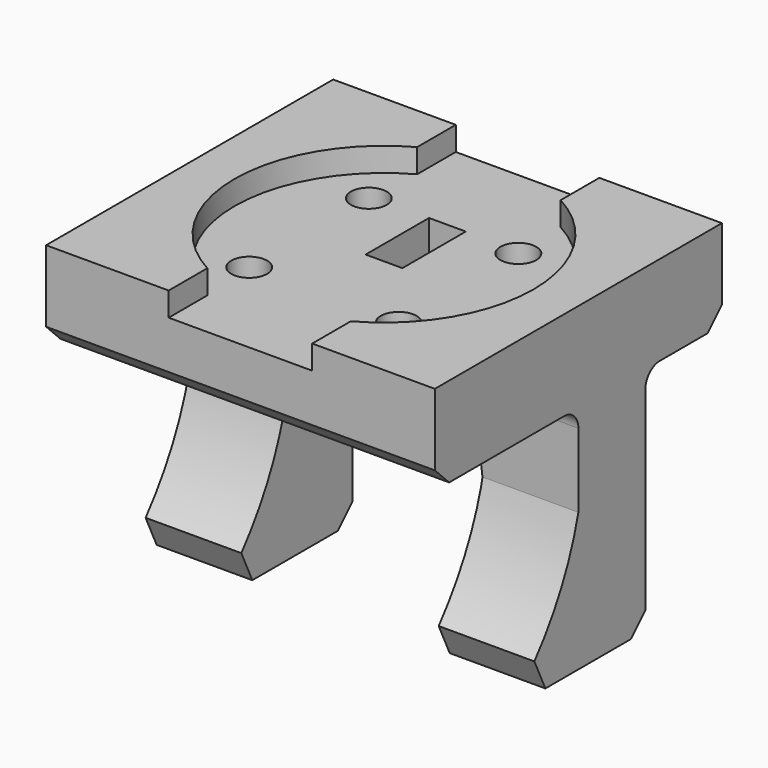
from build123d import *

# Parameters (mm, degrees)
F0_W          = 65
F0_H          = 60
F0_W_2        = 6.15
F0_H_2        = 13.25
F1_DEPTH      = 15
F3_DEPTH      = 14
F5_DEPTH      = 4
F6_R          = 3
F7_DEPTH      = 8
F9_DEPTH      = 90
F10_T4_DEPTH  = 29.425
F10_S5_R      = 16.5
F10_T6_DEPTH  = 16
F10_T10_DEPTH = 44.425
F10_S11_R     = 16.5
F10_T12_DEPTH = 24
F10_T17_DEPTH = 44.425
F10_S18_R     = 16.5
F10_T19_DEPTH = 24
F10_T24_DEPTH = 29.425
F10_S25_R     = 16.5
F10_T26_DEPTH = 16
F10_T30_DEPTH = 44.425
F10_S31_R     = 16.5
F10_T32_DEPTH = 24
F10_T37_DEPTH = 29.425
F10_S38_R     = 16.5
F10_T39_DEPTH = 16
F10_T43_DEPTH = 29.425
F10_S44_R     = 16.5
F10_T45_DEPTH = 16
F10_T49_DEPTH = 44.425
F10_S50_R     = 16.5
F10_T51_DEPTH = 24
F11_T1_DEPTH  = 80.4300979278
F11_T3_DEPTH  = 51.7830754439
F11_T5_DEPTH  = 51.7830754439
F11_T7_DEPTH  = 31.4300979278
F11_T9_DEPTH  = 31.4300979278


# Not quite as in the source:
# - a fillet or chamfer that OpenCascade refuses, or shapes differently, is made with other operations: its cross-section is extruded or revolved along the edge and cut away or added


with BuildPart() as f1:
    # F0 (on Top) → F1 (new body)
    with BuildSketch(Plane.XY):
        Rectangle(F0_W, F0_H)
        with Locations((0, 6.625)):
            Rectangle(F0_W_2, F0_H_2, mode=Mode.SUBTRACT)
    extrude(amount=F1_DEPTH)

    # F2 (on Front) → F3 (join, symmetric)
    with BuildSketch(Plane.XZ):
        with BuildLine():
            Line((-3.075, 0), (-32.5, 0))
            Line((-32.5, 0), (-32.5, -38.5))
            Line((-32.5, -38.5), (-16.5, -38.5))
            Line((-16.5, -38.5), (-16.5, -16.5))
            ThreePointArc((-16.5, -16.5), (-12.7080191218, -5.9759204678), (-3.075, -0.2890661898))
            Line((-3.075, -0.2890661898), (-3.075, 0))
        make_face()
        with BuildLine():
            Line((3.075, 0), (3.075, -0.2890661898))
            ThreePointArc((3.075, -0.2890661898), (12.7080191218, -5.9759204678), (16.5, -16.5))
            Line((16.5, -16.5), (16.5, -38.5))
            Line((16.5, -38.5), (32.5, -38.5))
            Line((32.5, -38.5), (32.5, 0))
            Line((32.5, 0), (3.075, 0))
        make_face()
    extrude(amount=F3_DEPTH, both=True)

    # F4 (on face) → F5 (cut)
    with BuildSketch(Plane.XY.offset(15)):
        with BuildLine():
            ThreePointArc((12, -21.9317121995), (25, 0), (12, 21.9317121995))
            Line((12, 21.9317121995), (12, 35))
            Line((12, 35), (-12, 35))
            Line((-12, 35), (-12, 21.9317121995))
            ThreePointArc((-12, 21.9317121995), (-25, 0), (-12, -21.9317121995))
            Line((-12, -21.9317121995), (-12, -35))
            Line((-12, -35), (12, -35))
            Line((12, -35), (12, -21.9317121995))
        make_face()
    extrude(amount=-F5_DEPTH, mode=Mode.SUBTRACT)

    # F6 (on face) → F7 (cut)
    with BuildSketch(Plane.XY.offset(11)):
        with Locations((-12.7, 12.7)):
            Circle(F6_R)
        with Locations((12.3, 12.7)):
            Circle(F6_R)
        with Locations((12.3, -12.3)):
            Circle(F6_R)
        with Locations((-12.7, -12.3)):
            Circle(F6_R)
    extrude(amount=-F7_DEPTH, mode=Mode.SUBTRACT)

    # F8 (on face) → F9 (cut)
    with BuildSketch(Plane.YZ.offset(32.5)):
        with BuildLine():
            Line((0, -15.3778724497), (0, 0))
            Line((0, 0), (-14, 0))
            Line((-14, 0), (-14, -38.5))
            ThreePointArc((-14, -38.5), (-5.2228777507, -28.0149492966), (0, -15.3778724497))
        make_face()
    extrude(amount=-F9_DEPTH, mode=Mode.SUBTRACT)

    # F10: fillet of radius 3 on 4 edges, made by hand


with BuildPart() as f10_tool2:
    # F10_s3 → F10_t4 (new body)
    with BuildSketch(Plane.YZ.offset(32.5)):
        with BuildLine():
            ThreePointArc((0, -3), (-0.8786796564, -0.8786796564), (-3, 0))
            Line((-3, 0), (0, 0))
            Line((0, 0), (0, -3))
        make_face()
    extrude(amount=-F10_T4_DEPTH)

    # F10_s5 → F10_t6 (cut, symmetric)
    with BuildSketch(Plane.XZ.offset(1.5)):
        with Locations((0, -16.5)):
            Circle(F10_S5_R)
    extrude(amount=F10_T6_DEPTH, both=True, mode=Mode.SUBTRACT)


with BuildPart() as f1_1:
    add(f1.part)

    # F10_t1: union F10_tool2
    add(f10_tool2.part)


with BuildPart() as f10_tool8:
    # F10_s9 → F10_t10 (new body)
    with BuildSketch(Plane.YZ.offset(40)):
        with BuildLine():
            ThreePointArc((0, -3), (-0.8786796564, -0.8786796564), (-3, 0))
            Line((-3, 0), (0, 0))
            Line((0, 0), (0, -3))
        make_face()
    extrude(amount=-F10_T10_DEPTH)

    # F10_s11 → F10_t12 (cut, symmetric)
    with BuildSketch(Plane.XZ.offset(1.5)):
        with Locations((0, -16.5)):
            Circle(F10_S11_R)
    extrude(amount=F10_T12_DEPTH, both=True, mode=Mode.SUBTRACT)

    split(bisect_by=Plane.YZ.offset(-3.075), keep=Keep.BOTTOM)


with BuildPart() as f1_2:
    add(f1_1.part)

    # F10_t7: union F10_tool8
    add(f10_tool8.part)


with BuildPart() as f10_tool15:
    # F10_s16 → F10_t17 (new body)
    with BuildSketch(Plane.YZ.offset(4.425)):
        with BuildLine():
            ThreePointArc((0, -3), (-0.8786796564, -0.8786796564), (-3, 0))
            Line((-3, 0), (0, 0))
            Line((0, 0), (0, -3))
        make_face()
    extrude(amount=-F10_T17_DEPTH)

    # F10_s18 → F10_t19 (cut, symmetric)
    with BuildSketch(Plane.XZ.offset(1.5)):
        with Locations((0, -16.5)):
            Circle(F10_S18_R)
    extrude(amount=F10_T19_DEPTH, both=True, mode=Mode.SUBTRACT)

    split(bisect_by=Plane.YZ.offset(3.075), keep=Keep.TOP)


with BuildPart() as f1_3:
    add(f1_2.part)

    # F10_t14: union F10_tool15
    add(f10_tool15.part)


with BuildPart() as f10_tool22:
    # F10_s23 → F10_t24 (new body)
    with BuildSketch(Plane.YZ.offset(-3.075)):
        with BuildLine():
            ThreePointArc((0, -3), (-0.8786796564, -0.8786796564), (-3, 0))
            Line((-3, 0), (0, 0))
            Line((0, 0), (0, -3))
        make_face()
    extrude(amount=-F10_T24_DEPTH)

    # F10_s25 → F10_t26 (cut, symmetric)
    with BuildSketch(Plane.XZ.offset(1.5)):
        with Locations((0, -16.5)):
            Circle(F10_S25_R)
    extrude(amount=F10_T26_DEPTH, both=True, mode=Mode.SUBTRACT)


with BuildPart() as f1_4:
    add(f1_3.part)

    # F10_t21: union F10_tool22
    add(f10_tool22.part)


with BuildPart() as f10_tool28:
    # F10_s29 → F10_t30 (new body)
    with BuildSketch(Plane.YZ.offset(4.425)):
        with BuildLine():
            ThreePointArc((14, -3), (14.8786796564, -0.8786796564), (17, 0))
            Line((17, 0), (14, 0))
            Line((14, 0), (14, -3))
        make_face()
    extrude(amount=-F10_T30_DEPTH)

    # F10_s31 → F10_t32 (cut, symmetric)
    with BuildSketch(Plane.XZ.offset(-15.5)):
        with Locations((0, -16.5)):
            Circle(F10_S31_R)
    extrude(amount=F10_T32_DEPTH, both=True, mode=Mode.SUBTRACT)

    split(bisect_by=Plane.YZ.offset(3.075), keep=Keep.TOP)


with BuildPart() as f1_5:
    add(f1_4.part)

    # F10_t27: union F10_tool28
    add(f10_tool28.part)


with BuildPart() as f10_tool35:
    # F10_s36 → F10_t37 (new body)
    with BuildSketch(Plane.YZ.offset(-3.075)):
        with BuildLine():
            ThreePointArc((14, -3), (14.8786796564, -0.8786796564), (17, 0))
            Line((17, 0), (14, 0))
            Line((14, 0), (14, -3))
        make_face()
    extrude(amount=-F10_T37_DEPTH)

    # F10_s38 → F10_t39 (cut, symmetric)
    with BuildSketch(Plane.XZ.offset(-15.5)):
        with Locations((0, -16.5)):
            Circle(F10_S38_R)
    extrude(amount=F10_T39_DEPTH, both=True, mode=Mode.SUBTRACT)


with BuildPart() as f1_6:
    add(f1_5.part)

    # F10_t34: union F10_tool35
    add(f10_tool35.part)


with BuildPart() as f10_tool41:
    # F10_s42 → F10_t43 (new body)
    with BuildSketch(Plane.YZ.offset(32.5)):
        with BuildLine():
            ThreePointArc((14, -3), (14.8786796564, -0.8786796564), (17, 0))
            Line((17, 0), (14, 0))
            Line((14, 0), (14, -3))
        make_face()
    extrude(amount=-F10_T43_DEPTH)

    # F10_s44 → F10_t45 (cut, symmetric)
    with BuildSketch(Plane.XZ.offset(-15.5)):
        with Locations((0, -16.5)):
            Circle(F10_S44_R)
    extrude(amount=F10_T45_DEPTH, both=True, mode=Mode.SUBTRACT)


with BuildPart() as f1_7:
    add(f1_6.part)

    # F10_t40: union F10_tool41
    add(f10_tool41.part)


with BuildPart() as f10_tool47:
    # F10_s48 → F10_t49 (new body)
    with BuildSketch(Plane.YZ.offset(40)):
        with BuildLine():
            ThreePointArc((14, -3), (14.8786796564, -0.8786796564), (17, 0))
            Line((17, 0), (14, 0))
            Line((14, 0), (14, -3))
        make_face()
    extrude(amount=-F10_T49_DEPTH)

    # F10_s50 → F10_t51 (cut, symmetric)
    with BuildSketch(Plane.XZ.offset(-15.5)):
        with Locations((0, -16.5)):
            Circle(F10_S50_R)
    extrude(amount=F10_T51_DEPTH, both=True, mode=Mode.SUBTRACT)

    split(bisect_by=Plane.YZ.offset(-3.075), keep=Keep.BOTTOM)


with BuildPart() as f1_8:
    add(f1_7.part)

    # F10_t46: union F10_tool47
    add(f10_tool47.part)

    # F11: chamfer of 3 on 6 edges, made by hand

    # F11_s2 → F11_t1 (cut)
    with BuildSketch(Plane.YZ.offset(-40.2150489639)):
        Polygon((-30, 3), (-27, 0), (-30, 0), align=None)
        Polygon((27, 0), (30, 3), (30, 0), align=None)
    extrude(amount=F11_T1_DEPTH, mode=Mode.SUBTRACT)

    # F11_s4 → F11_t3 (cut)
    with BuildSketch(Plane.YZ.offset(-50.391537722)):
        with BuildLine():
            Line((-6.8950157601, -38.5), (-9.1963693219, -33.5754814152))
            ThreePointArc((-9.1963693219, -33.5754814152), (-11.4890994339, -36.1144458386), (-14, -38.5))
            Line((-14, -38.5), (-6.8950157601, -38.5))
        make_face()
    extrude(amount=F11_T3_DEPTH, mode=Mode.SUBTRACT)

    # F11_s6 → F11_t5 (cut)
    with BuildSketch(Plane.YZ.offset(-1.391537722)):
        with BuildLine():
            Line((-9.1963693219, -33.5754814152), (-6.8950157601, -38.5))
            Line((-6.8950157601, -38.5), (-14, -38.5))
            ThreePointArc((-14, -38.5), (-11.4890994339, -36.1144458386), (-9.1963693219, -33.5754814152))
        make_face()
    extrude(amount=F11_T5_DEPTH, mode=Mode.SUBTRACT)

    # F11_s8 → F11_t7 (cut)
    with BuildSketch(Plane.YZ.offset(8.7849510361)):
        Polygon((11, -38.5), (14, -35.5), (14, -38.5), align=None)
    extrude(amount=F11_T7_DEPTH, mode=Mode.SUBTRACT)

    # F11_s10 → F11_t9 (cut)
    with BuildSketch(Plane.YZ.offset(-40.2150489639)):
        Polygon((11, -38.5), (14, -35.5), (14, -38.5), align=None)
    extrude(amount=F11_T9_DEPTH, mode=Mode.SUBTRACT)


solid = f1_8.part
